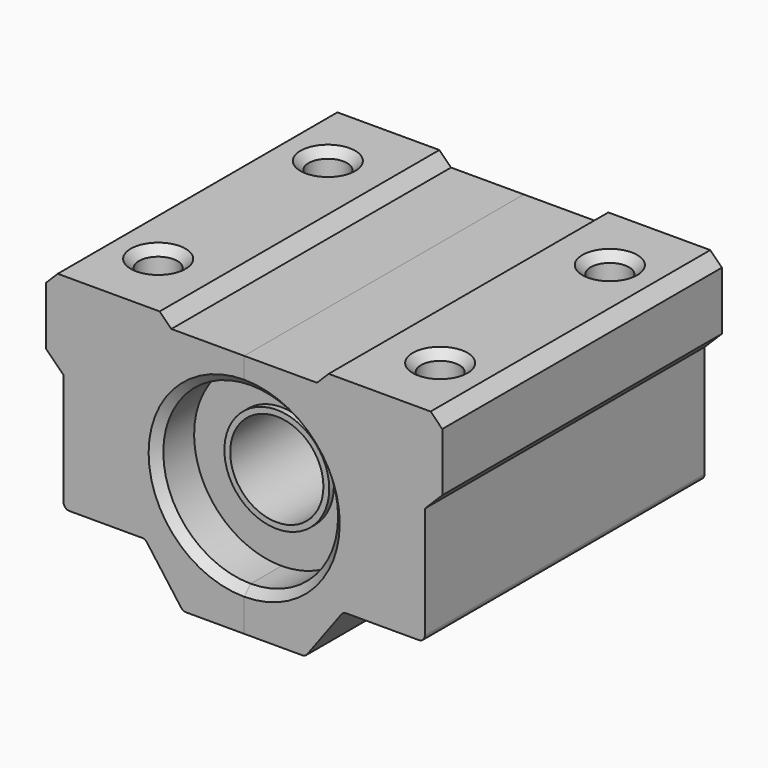
from build123d import *
from build123d import SkipClean  # not in build123d's __all__

# Parameters (mm, degrees)
F1_DEPTH       = 15
F2_SIZE        = 0.99999
F3_SIZE        = 1.49999
F4_R           = 0.5
F6_D           = 3
F6_CBORE_D     = 3.3
F6_CBORE_DEPTH = 6
F7_SIZE        = 0.7
F0_R           = 4.5
F8_DEPTH       = 11
F0_R_2         = 4
F9_DEPTH       = 11.5


# Not quite as in the source:
# - a fillet or chamfer is up to 0.001 mm smaller than in the source, because OpenCascade refuses the exact size


with BuildPart() as f1:
    # F0 (on Front) → F1 (new body, symmetric)
    with BuildSketch(Plane.XZ):
        with BuildLine():
            ThreePointArc((0, 7.5), (5.3033008589, 5.3033008589), (7.5, 0))
            ThreePointArc((7.5, 0), (5.3033008589, -5.3033008589), (0, -7.5))
            Line((0, -7.5), (0, -11))
            Line((0, -11), (5.25, -11))
            Line((5.25, -11), (8.5, -6.6))
            Line((8.5, -6.6), (15.5, -6.6))
            Line((15.5, -6.6), (15.5, 3.5))
            Line((15.5, 3.5), (17, 3.5))
            Line((17, 3.5), (17, 11))
            Line((17, 11), (7.25, 11))
            Line((7.25, 11), (7.25, 10))
            Line((7.25, 10), (0, 10))
            Line((0, 10), (0, 7.5))
        make_face()
    extrude(amount=F1_DEPTH, both=True)

    # F2 (size 1 in the source; OpenCascade refuses exactly that, so slightly less here)
    f2_edges = [f1.edges().sort_by_distance(p)[0] for p in [
        (7.25, 0, 10),
        (17, 0, 11),
    ]]
    chamfer(f2_edges, length=F2_SIZE)

    # F3 (size 1.5 in the source; OpenCascade refuses exactly that, so slightly less here)
    f3_edges = [f1.edges().sort_by_distance(p)[0] for p in [
        (17, 0, 3.5),
    ]]
    chamfer(f3_edges, length=F3_SIZE)

    # F4
    f4_edges = [f1.edges().sort_by_distance(p)[0] for p in [
        (15.5, 0, -6.6),
        (8.5, 0, -6.6),
        (5.25, 0, -11),
    ]]
    fillet(f4_edges, radius=F4_R)

    # F6 (through all)
    with Locations(Plane.XY.offset(11)):
        with Locations((12.1, 9.1), (12.1, -9.1)):
            CounterBoreHole(F6_D / 2, F6_CBORE_D / 2, F6_CBORE_DEPTH)

    # F7
    f7_edges = [f1.edges().sort_by_distance(p)[0] for p in [
        (7.5, -15, 0),
        (7.5, 15, 0),
        (10.45, 9.1, 11),
        (10.45, -9.1, 11),
    ]]
    chamfer(f7_edges, length=F7_SIZE)

    # F10: F1 across plane


with BuildPart() as f8:
    # F0 (on Front) → F8 (new body, symmetric)
    with BuildSketch(Plane.XZ):
        with BuildLine():
            ThreePointArc((0, -7.5), (5.3033008589, -5.3033008589), (7.5, 0))
            ThreePointArc((7.5, 0), (5.3033008589, 5.3033008589), (0, 7.5))
            ThreePointArc((0, 7.5), (-7.5, 0), (0, -7.5))
        make_face()
        Circle(F0_R, mode=Mode.SUBTRACT)
    extrude(amount=F8_DEPTH, both=True)

    # F0 (on Front) → F9 (join, symmetric)
    with BuildSketch(Plane.XZ):
        Circle(F0_R)
        Circle(F0_R_2, mode=Mode.SUBTRACT)
    extrude(amount=F9_DEPTH, both=True)


with BuildPart() as f1_1:
    add(f1.part, clean=False)
    with SkipClean():  # cleaning this boolean's faces spoils the solid; the shape is the same uncleaned
        add(f1.part.mirror(Plane.YZ), clean=False)


solid = Compound([f8.part, f1_1.part])
